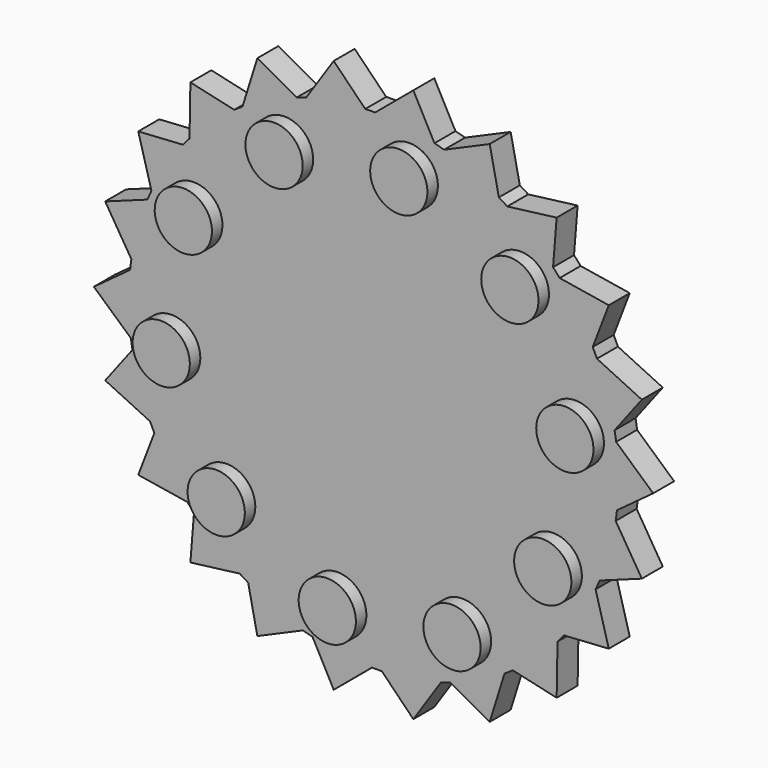
from build123d import *

# Parameters (mm, degrees)
F0_R            = 118.6771656213
F1_DEPTH        = 6.35
F2_R            = 13.8727461935
F3_DEPTH        = 6.35
F3_COPIES_COUNT = 10
F5_DEPTH        = 12.7
F5_COPIES_COUNT = 22


# Not quite as in the source:
# - a pattern or mirror of a feature is missing from the dataset's text; its kind, count and spacing are read off the source's solid


with BuildPart() as f1:
    # F0 (on Front) → F1 (new body, symmetric)
    with BuildSketch(Plane.XZ):
        Circle(F0_R)
    extrude(amount=F1_DEPTH, both=True)

    # F2 (on face) → F3 (join)
    with BuildSketch(Plane.XZ.offset(6.35)):
        with Locations((-71.153357625, -68.4610754251)):
            Circle(F2_R)
    f3 = extrude(amount=F3_DEPTH)

    # F3_copies: F3 ×10 about axis
    f3_copies_axis = Axis((0, 0, 0), (0, 1, 0))
    for i in range(1, F3_COPIES_COUNT):
        add(f3.rotate(f3_copies_axis, i * 360 / F3_COPIES_COUNT))

    # F4 (on face) → F5 (join, through all)
    with BuildSketch(Plane.XZ.offset(6.35)):
        with BuildLine():
            Line((-135.5267614126, 0), (-117.5784646417, -16.1113094564))
            ThreePointArc((-117.5784646417, -16.1113094564), (-118.6661963279, -1.6135330732), (-117.9730534673, 12.9084582934))
            Line((-117.9730534673, 12.9084582934), (-135.5267614126, 0))
        make_face()
    f5 = extrude(amount=-F5_DEPTH)

    # F5_copies: F5 ×22 about axis
    f5_copies_axis = Axis((0, 0, 0), (0, 1, 0))
    for i in range(1, F5_COPIES_COUNT):
        add(f5.rotate(f5_copies_axis, i * 360 / F5_COPIES_COUNT))


solid = f1.part
